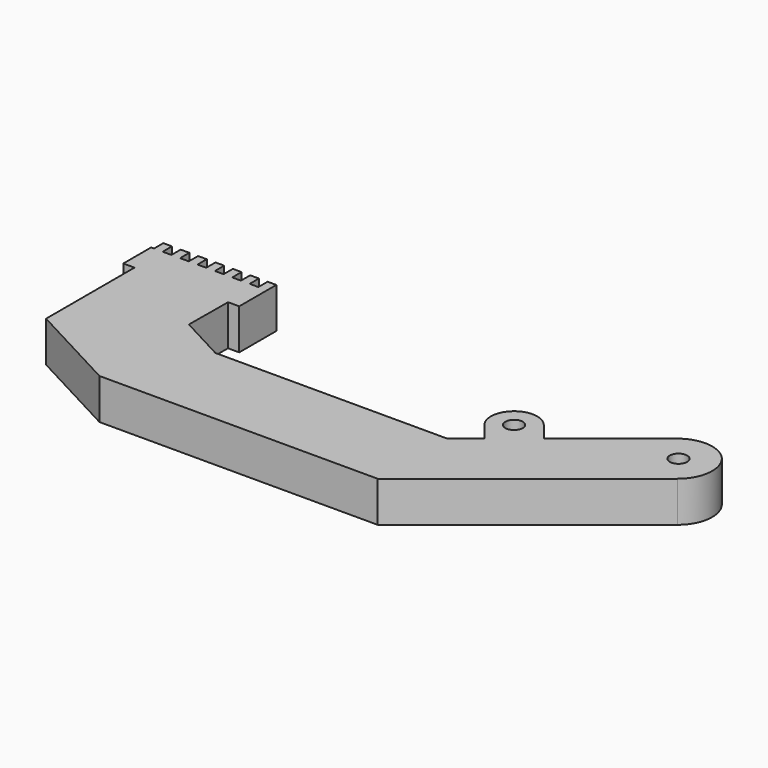
from build123d import *

# Parameters (mm, degrees)
F0_R        = 1.5
F1_DEPTH    = 7
F2_R        = 3.99999
F3_T1_DEPTH = 37
F4_W        = 20
F4_H        = 7
F5_DEPTH    = 6
F6_W        = 1.5
F6_H        = 7
F7_DEPTH    = 2


# Not quite as in the source:
# - a fillet or chamfer that OpenCascade refuses, or shapes differently, is made with other operations: its cross-section is extruded or revolved along the edge and cut away or added
# - a fillet or chamfer is up to 0.001 mm smaller than in the source, because OpenCascade refuses the exact size


with BuildPart() as f1:
    # F0 (on Top) → F1 (new body)
    with BuildSketch(Plane.XY):
        Polygon((-79.2163482308, -9.9173756316), (-95.3576945582, -9.9173756316), (-95.3576945582, -28.9785558952), (-79.2939967774, -37.5458613783), (-31.2939967774, -37.5458613783), (4.9152223427, -8.5784860822), (-2.401850828, 0.5678553812), (-21.1427022546, -14.4248257601), (-26.1402626351, -8.1778752846), (-32.3872131106, -13.175435665), (-27.3896527302, -19.4223861405), (-31.2939967774, -22.5458613783), (-71.2939967774, -22.5458613783), (-79.2678481488, -18.2931406469), align=None)
        with Locations((-26.7649576826, -13.8001307126)):
            Circle(F0_R, mode=Mode.SUBTRACT)
        with Locations((-3.3164724251, -7.6638418965)):
            Circle(F0_R, mode=Mode.SUBTRACT)
    extrude(amount=F1_DEPTH)

    # F2 (radius 4 in the source; OpenCascade refuses exactly that, so slightly less here)
    f2_edges = [f1.edges().sort_by_distance(p)[0] for p in [
        (-26.140263, -8.177875, 3.5),
        (-32.387213, -13.175436, 3.5),
    ]]
    fillet(f2_edges, radius=F2_R)

    # F3: fillet of radius 6 on 2 edges, made by hand

    # F3_s2 → F3_t1 (cut)
    with BuildSketch(Plane.XY.offset(-15)):
        with BuildLine():
            ThreePointArc((-7.0870636847, -3.1803149041), (-2.6763042429, -1.9022253527), (1.3463194573, -4.1173574755))
            Line((1.3463194573, -4.1173574755), (-2.401850828, 0.5678553812))
            Line((-2.401850828, 0.5678553812), (-7.0870636847, -3.1803149041))
        make_face()
        with BuildLine():
            ThreePointArc((1.1670520574, -3.8932732256), (2.4451416088, -8.3040326673), (0.2300094861, -12.3266563675))
            Line((0.2300094861, -12.3266563675), (4.9152223427, -8.5784860822))
            Line((4.9152223427, -8.5784860822), (1.1670520574, -3.8932732256))
        make_face()
    extrude(amount=F3_T1_DEPTH, mode=Mode.SUBTRACT)

    # F4 (on face) → F5 (join)
    with BuildSketch(Plane(origin=(0, -9.9173756316, 0), x_dir=(-1, 0, 0), z_dir=(0, 1, 0))):
        with Locations((87.2870213945, 3.5)):
            Rectangle(F4_W, F4_H)
    extrude(amount=F5_DEPTH)

    # F6 (on face) → F7 (join)
    with BuildSketch(Plane(origin=(0, -3.9173756316, 0), x_dir=(-1, 0, 0), z_dir=(0, 1, 0))):
        with Locations((78.0370213945, 3.5)):
            Rectangle(F6_W, F6_H)
        with Locations((81.0370213945, 3.5)):
            Rectangle(F6_W, F6_H)
        with Locations((84.0370213945, 3.5)):
            Rectangle(F6_W, F6_H)
        with Locations((87.0370213945, 3.5)):
            Rectangle(F6_W, F6_H)
        with Locations((90.0370213945, 3.5)):
            Rectangle(F6_W, F6_H)
        with Locations((93.0370213945, 3.5)):
            Rectangle(F6_W, F6_H)
        with Locations((96.0370213945, 3.5)):
            Rectangle(F6_W, F6_H)
    extrude(amount=F7_DEPTH)


solid = f1.part
